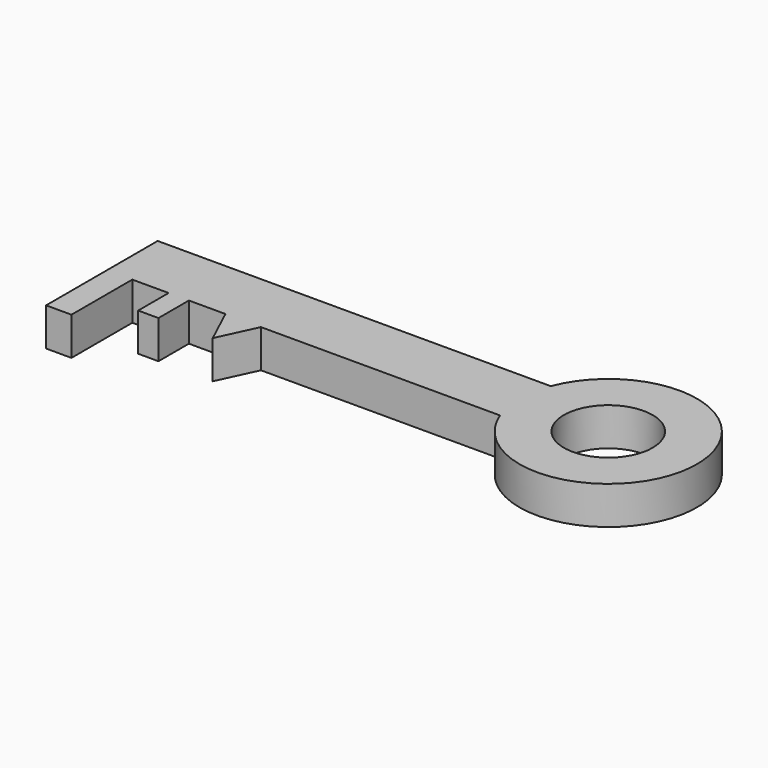
from build123d import *

# Parameters (mm, degrees)
F0_R     = 17.5
F0_W     = 10
F0_H     = 30
F0_W_2   = 8
F0_H_2   = 15
F1_DEPTH = 15


# Not quite as in the source:
# - a feature of the source that left no trace in its solid (it failed there, or was rolled back) is left out


with BuildPart() as f1:
    # F0 (on Top) → F1 (new body)
    with BuildSketch(Plane.XY):
        Polygon((-94.275398612, 0), (0, 0), (0, 25), (-155, 25), (-155, 0), (-145, 0), (-130.6804269552, 0), (-122.6804269552, 0), (-108.275398612, 0), align=None)
        with BuildLine():
            Line((0, 25), (0, 0))
            ThreePointArc((0, 0), (67.6917420766, 12.5), (0, 25))
        make_face()
        with Locations((32.6917420766, 12.5)):
            Circle(F0_R, mode=Mode.SUBTRACT)
        with Locations((-150, -15)):
            Rectangle(F0_W, F0_H)
        with Locations((-126.6804269552, -7.5)):
            Rectangle(F0_W_2, F0_H_2)
        Polygon((-101.275398612, -15), (-94.275398612, 0), (-108.275398612, 0), align=None)
    extrude(amount=F1_DEPTH)


solid = f1.part
